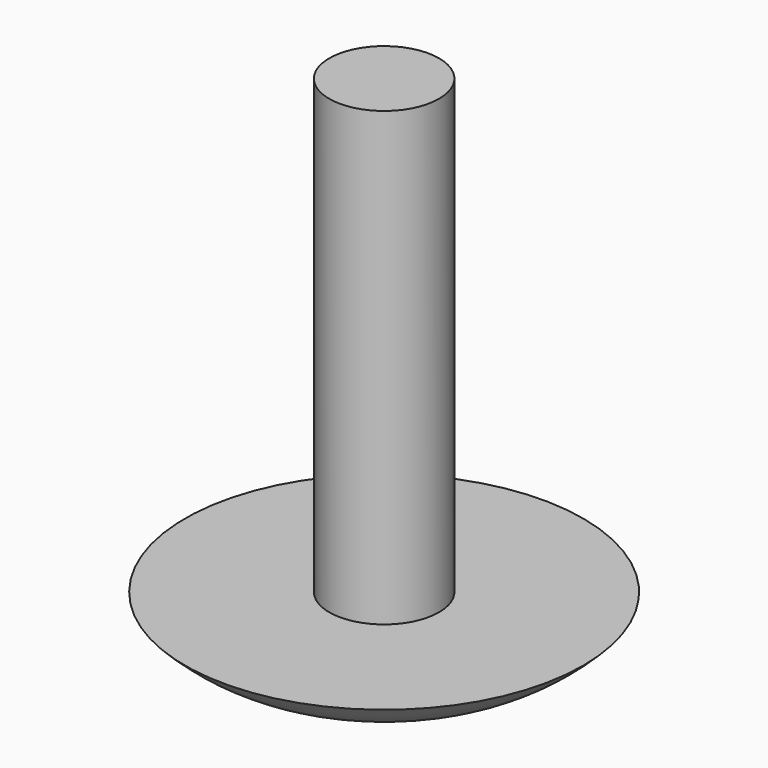
from build123d import *

# Parameters (mm, degrees)
F0_R     = 9.25
F1_DEPTH = 2.7
F2_R     = 2.55
F3_DEPTH = 21


# Not quite as in the source:
# - a fillet or chamfer that OpenCascade refuses, or shapes differently, is made with other operations: its cross-section is extruded or revolved along the edge and cut away or added


with BuildPart() as f1:
    # F0 (on Top) → F1 (new body)
    with BuildSketch(Plane.XY):
        Circle(F0_R)
    extrude(amount=F1_DEPTH)

    # F2 (on face) → F3 (join)
    with BuildSketch(Plane.XY.offset(2.7)):
        Circle(F2_R)
    extrude(amount=F3_DEPTH)

    # F4: fillet of radius 9 on 1 edges, made by hand

    # F4_s1 → F4_t2 (revolve, cut)
    with BuildSketch(Plane.XZ):
        with BuildLine():
            ThreePointArc((9.25, 2.7), (6.3083994259, 0.7024099884), (2.8227144143, 0))
            Line((2.8227144143, 0), (9.25, 0))
            Line((9.25, 0), (9.25, 2.7))
        make_face()
    revolve(axis=Axis((0, 0, 0), (0, 0, 1)), mode=Mode.SUBTRACT)


solid = f1.part
